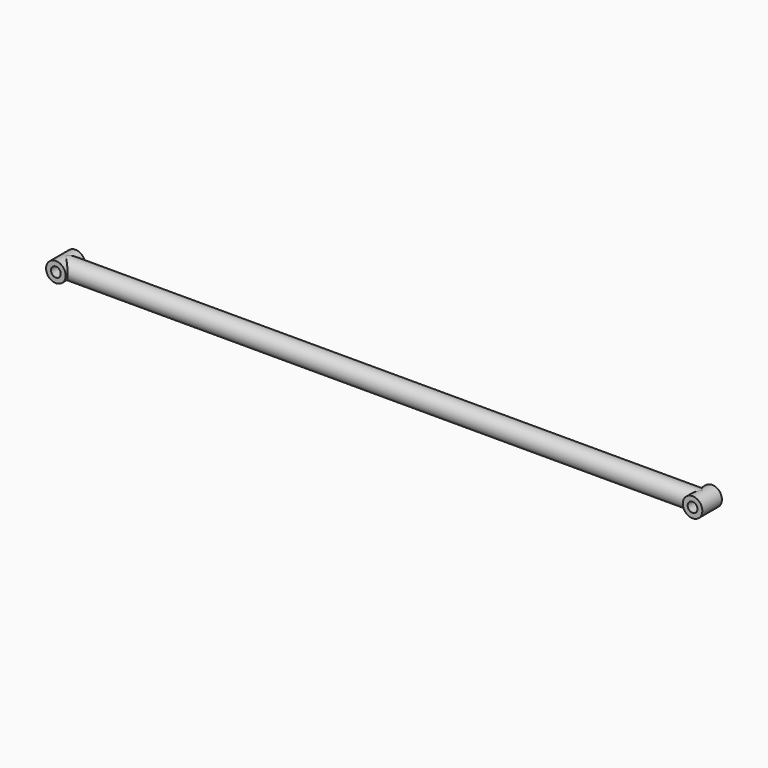
from build123d import *

# Parameters (mm, degrees)
F1_DEPTH      = 15.875
F0_R          = 12.7
F3_END_RADIUS = 12.7
F2_R          = 12.7
F3_REACH      = 874.1220244843
F7_R          = 6.35
F8_DEPTH      = 50.8


# Not quite as in the source:
# - a feature of the source that left no trace in its solid (it failed there, or was rolled back) is left out


with BuildPart() as f1:
    # F0 (on Front) → F1 (new body, symmetric)
    with BuildSketch(Plane.XZ):
        with BuildLine():
            ThreePointArc((838.2, 0), (825.5, 12.7), (812.8, 0))
            ThreePointArc((812.8, 0), (825.5, -12.7), (838.2, 0))
        make_face()
        with BuildLine():
            ThreePointArc((819.15, 0), (825.5, 6.35), (831.85, 0))
            ThreePointArc((831.85, 0), (825.5, -6.35), (819.15, 0))
        make_face(mode=Mode.SUBTRACT)
    extrude(amount=F1_DEPTH, both=True)



with BuildPart() as f1b:
    # F0 (on Front) → F1, piece 2 (new body, symmetric)
    with BuildSketch(Plane.XZ):
        Circle(F0_R)
    extrude(amount=F1_DEPTH, both=True)


with BuildPart() as f1_1:
    add(f1.part)

    add(f1b.part)  # F3 merges F1b
    f3_end = (Plane(origin=(825.5, 7.9375, 0), x_dir=(0, 0, -1), z_dir=(0, -1, 0)) * Cylinder(F3_END_RADIUS, 3451.9858515901, mode=Mode.PRIVATE)).faces().sort_by_distance((825.5, 7.9375, 12.7))[0]
    # F2 (on Right) → F3 (join, up to the whole of a round face its end follows)
    with BuildSketch(Plane.YZ):
        Circle(F2_R)
    f3_long = extrude(amount=F3_REACH, mode=Mode.PRIVATE)
    add(split(f3_long, bisect_by=f3_end, keep=Keep.ALL, mode=Mode.PRIVATE).solids().sort_by_distance((0, 0, 0))[0])

    # F7 (on face) → F8 (cut)
    with BuildSketch(Plane.XZ.offset(15.875)):
        Circle(F7_R)
    extrude(amount=-F8_DEPTH, mode=Mode.SUBTRACT)


solid = f1_1.part
